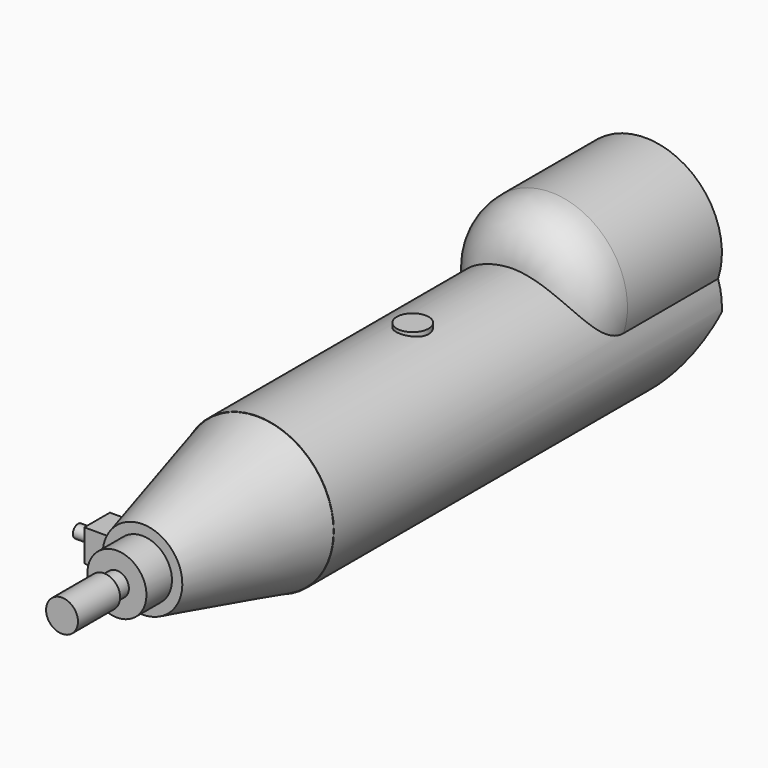
from build123d import *

# Parameters (mm, degrees)
F0_R      = 24
F1_DEPTH  = 152
F2_R      = 24
F3_DEPTH  = 52
F6_W      = 10
F6_H      = 9.25
F10_W     = 10
F10_H     = 10
F11_DEPTH = 19
F12_R     = 2
F13_DEPTH = 6
F15_DEPTH = 30
F16_W     = 11.4625198767
F16_H     = 18.1046463549
F17_DEPTH = 2
F18_ANGLE = 90
F19_R     = 5
F20_DEPTH = 25
F21_W     = 4.3103364494
F21_H     = 12.3563234784
F22_DEPTH = 25
F23_R     = 14.99999


# Not quite as in the source:
# - a fillet or chamfer is up to 0.001 mm smaller than in the source, because OpenCascade refuses the exact size


with BuildPart() as f1:
    # F0 (on Front) → F1 (new body)
    with BuildSketch(Plane.XZ):
        Circle(F0_R)
    extrude(amount=F1_DEPTH)

    # F2 (on Front) → F3 (join)
    with BuildSketch(Plane.XZ):
        with Locations((0, 15)):
            Circle(F2_R)
    extrude(amount=F3_DEPTH)

    # F4 (on Right) → F5 (revolve)
    with BuildSketch(Plane.YZ):
        Polygon((-197, 0), (-152, 0), (-151.5667739129, 23.9960895805), (-197, 12.5), align=None)
    revolve(axis=Axis((0, -174.5, 0), (0, -1, 0)))

    # F6 (on Right) → F7 (revolve)
    with BuildSketch(Plane.YZ):
        with Locations((-202, 4.625)):
            Rectangle(F6_W, F6_H)
    revolve(axis=Axis((0, -202, 0), (0, -1, 0)))

    # F8 (on Right) → F9 (revolve)
    with BuildSketch(Plane.YZ):
        Polygon((-228.5, 0), (-207, 0), (-207, 3.75), (-212, 3.75), (-212, 5), (-228.5, 5), align=None)
    revolve(axis=Axis((0, -217.75, 0), (0, -1, 0)))

    # F14 (on Right) → F15 (cut, symmetric)
    with BuildSketch(Plane.YZ):
        Polygon((-23, -24.3253242224), (0, -24.3253242224), (0, -1.3253242224), align=None)
    extrude(amount=F15_DEPTH, both=True, mode=Mode.SUBTRACT)



with BuildPart() as f11:
    # F10 (on Top) → F11 (new body)
    with BuildSketch(Plane.XY):
        with Locations((0, -191)):
            Rectangle(F10_W, F10_H)
    extrude(amount=-F11_DEPTH)


with BuildPart() as f13:
    # F12 (on face) → F13 (new body)
    with BuildSketch(Plane(origin=(0, 0, -19), x_dir=(1, 0, 0), z_dir=(0, 0, -1))):
        with Locations((0, 191)):
            Circle(F12_R)
    extrude(amount=F13_DEPTH)


with BuildPart() as f17:
    # F16 (on face) → F17 (new body)
    with BuildSketch(Plane(origin=(0, 0.6626621112, -0.6626621112), x_dir=(-1, 0, 0), z_dir=(0, 0.7071067812, -0.7071067812))):
        with Locations((0, -15.9248393029)):
            Rectangle(F16_W, F16_H)
    extrude(amount=F17_DEPTH)


with BuildPart() as f11_1:
    # F18: moved
    add(f11.part.rotate(Axis((0, 0, 0), (0, 1, 0)), F18_ANGLE))


with BuildPart() as f13_1:
    # F18: moved
    add(f13.part.rotate(Axis((0, 0, 0), (0, 1, 0)), F18_ANGLE))


with BuildPart() as f20:
    # F19 (on Top) → F20 (new body, symmetric)
    with BuildSketch(Plane.XY):
        with Locations((0, -91.1234393716)):
            Circle(F19_R)
    extrude(amount=F20_DEPTH, both=True)


with BuildPart() as f1_1:
    add(f1.part)

    add(f11_1.part)  # F22 merges F11

    add(f13_1.part)  # F22 merges F13

    add(f17.part)  # F22 merges F17

    add(f20.part)  # F22 merges F20
    # F21 (on Top) → F22 (join)
    with BuildSketch(Plane.XY):
        with Locations((0, -43.8218382608)):
            Rectangle(F21_W, F21_H)
    extrude(amount=-F22_DEPTH)

    # F23 (radius 15 in the source; OpenCascade refuses exactly that, so slightly less here)
    f23_edges = [f1_1.edges().sort_by_distance(p)[0] for p in [
        (0, -52, 39),
    ]]
    fillet(f23_edges, radius=F23_R)


solid = f1_1.part
